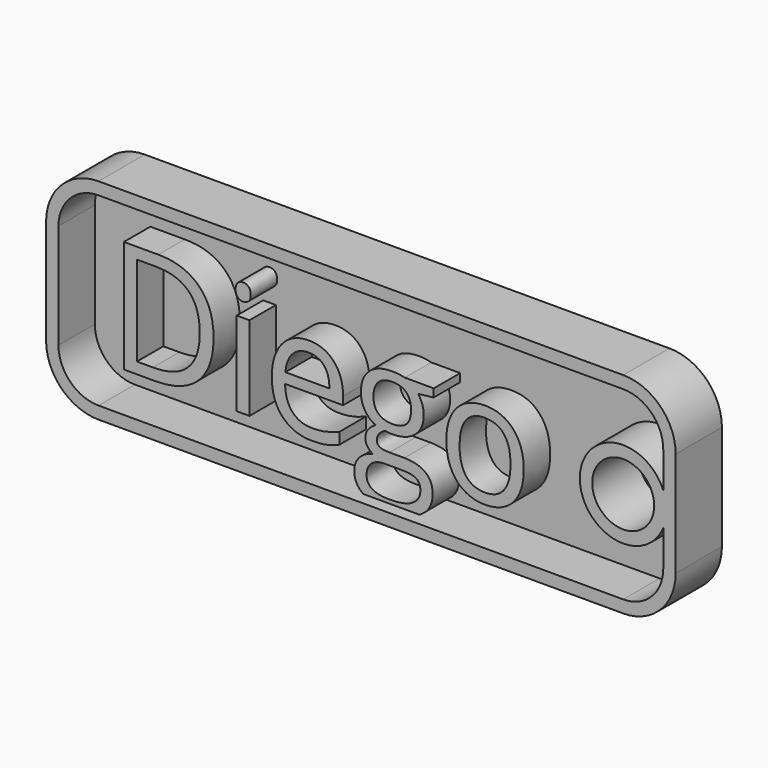
from build123d import *

# Parameters (mm, degrees)
F0_R         = 3.75
F1_DEPTH     = 7
F2_T         = -1.5
F3_TEXT_SIZE = 19.0472593562
F4_DEPTH     = 4


# Not quite as in the source:
# - Text() gives the source's letters only with a copy of the font that has no kerning and outlines rounded to 1/6400 em; it was checked with that copy


with BuildPart() as f1:
    # F0 (on Front) → F1 (new body)
    with BuildSketch(Plane.XZ):
        with BuildLine():
            ThreePointArc((38.1, 6.35), (36.2401280605, 10.8401280605), (31.75, 12.7))
            Line((31.75, 12.7), (-31.75, 12.7))
            ThreePointArc((-31.75, 12.7), (-36.2401280605, 10.8401280605), (-38.1, 6.35))
            Line((-38.1, 6.35), (-38.1, -6.35))
            ThreePointArc((-38.1, -6.35), (-36.2401280605, -10.8401280605), (-31.75, -12.7))
            Line((-31.75, -12.7), (31.75, -12.7))
            ThreePointArc((31.75, -12.7), (36.2401280605, -10.8401280605), (38.1, -6.35))
            Line((38.1, -6.35), (38.1, 6.35))
        make_face()
        with Locations((31.75, 0)):
            Circle(F0_R, mode=Mode.SUBTRACT)
    extrude(amount=F1_DEPTH)

    # F2
    f2_openings = [f1.faces().sort_by_distance(p)[0] for p in [
        (-0.75547, -7, 0),
    ]]
    offset(amount=F2_T, openings=f2_openings)

    # F3 (on face) → F4 (join)
    with BuildSketch(Plane.XZ.offset(1.5)):
        with Locations((-31.75, -7.3640267365)):
            Text('Diego', F3_TEXT_SIZE, font='Open Sans', text_align=(TextAlign.LEFT, TextAlign.BOTTOM))
    extrude(amount=F4_DEPTH)


solid = f1.part
